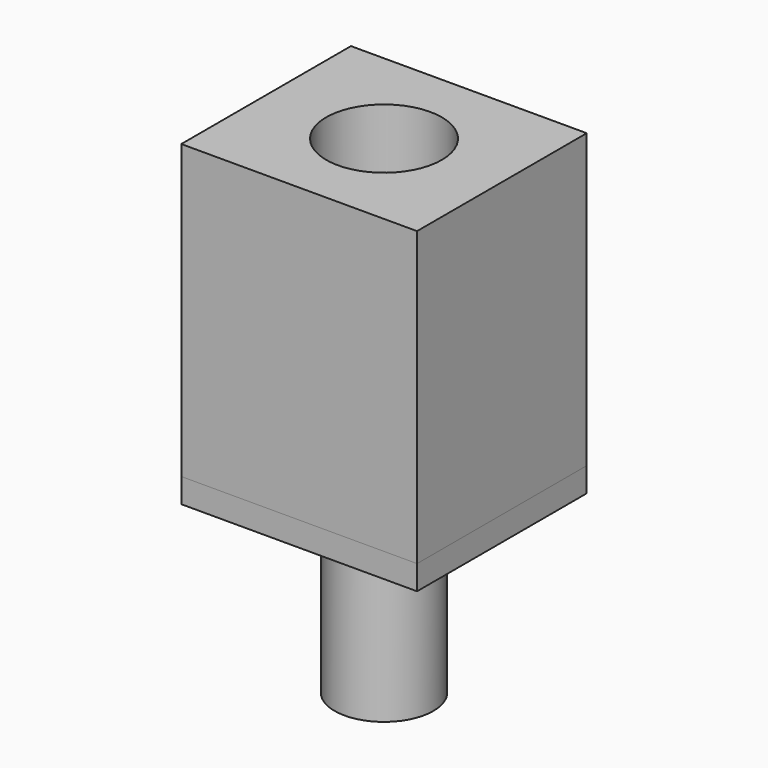
from build123d import *

# Parameters (mm, degrees)
F0_W     = 61.3812096417
F0_H     = 55.2162826061
F0_R     = 15.0467047404
F1_DEPTH = 76.2
F0_R_2   = 12.8526590503
F2_DEPTH = 50.8
F3_DEPTH = 6.35


with BuildPart() as f1:
    # F0 (on Top) → F1 (new body)
    with BuildSketch(Plane.XY):
        Rectangle(F0_W, F0_H)
        Circle(F0_R, mode=Mode.SUBTRACT)
    extrude(amount=F1_DEPTH)


with BuildPart() as f2:
    # F0 (on Top) → F2 (new body)
    with BuildSketch(Plane.XY):
        Circle(F0_R_2)
    extrude(amount=-F2_DEPTH)

    # F0 (on Top) → F3 (join)
    with BuildSketch(Plane.XY):
        Rectangle(F0_W, F0_H)
        Circle(F0_R, mode=Mode.SUBTRACT)
        Circle(F0_R)
        Circle(F0_R_2, mode=Mode.SUBTRACT)
    extrude(amount=-F3_DEPTH)


solid = Compound([f1.part, f2.part])
